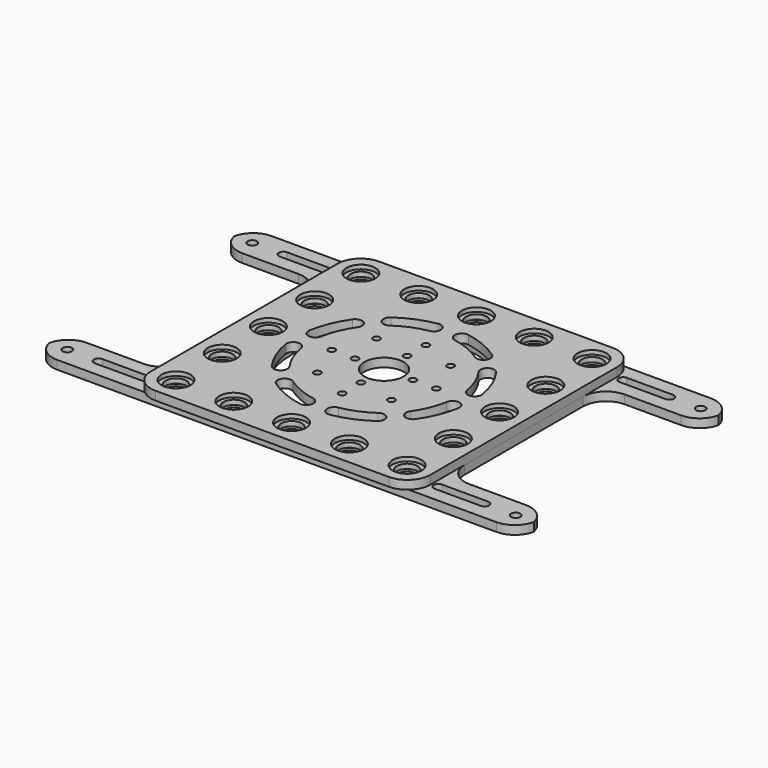
from build123d import *

# Parameters (mm, degrees)
F0_R        = 4.5
F0_W        = 24
F0_H        = 4
F0_R_2      = 2
F1_DEPTH    = 3.75
F2_T1_DEPTH = 3.75
F2_T3_DEPTH = 53.75
F3_R        = 2.5
F4_R        = 1.99999
F9_W        = 121
F9_H        = 121
F9_R        = 6.25
F9_R_2      = 1.5
F9_R_3      = 8.5
F10_DEPTH   = 3.75
F9_R_4      = 4.5
F11_DEPTH   = 2
F12_R       = 10
F6_R        = 6.25
F6_R_2      = 4.5
F13_DEPTH   = 1


# Not quite as in the source:
# - a fillet or chamfer that OpenCascade refuses, or shapes differently, is made with other operations: its cross-section is extruded or revolved along the edge and cut away or added
# - two fillets or chamfers of one size are made in one step
# - a fillet or chamfer is up to 0.001 mm smaller than in the source, because OpenCascade refuses the exact size
# - a feature names something its author has since deleted; it is built from what else it names


with BuildPart() as f1:
    # F0 (on Top) → F1 (new body)
    with BuildSketch(Plane.XY):
        with BuildLine():
            ThreePointArc((28.2842712475, 28.2842712475), (36.9551813005, 15.3073372946), (40, 0))
            ThreePointArc((40, 0), (28.2842712475, -28.2842712475), (0, -40))
            Line((0, -40), (0, -45.5))
            ThreePointArc((0, -45.5), (3.1819805153, -46.8180194847), (4.5, -50))
            ThreePointArc((4.5, -50), (3.1819805153, -53.1819805153), (0, -54.5))
            Line((0, -54.5), (0, -58))
            Line((0, -58), (105, -58))
            Line((105, -58), (105, -42))
            Line((105, -42), (60.5, -42))
            Line((60.5, -42), (60.5, 42))
            Line((60.5, 42), (105, 42))
            Line((105, 42), (105, 58))
            Line((105, 58), (0, 58))
            Line((0, 58), (0, 54.5))
            ThreePointArc((0, 54.5), (3.1819805153, 53.1819805153), (4.5, 50))
            ThreePointArc((4.5, 50), (3.1819805153, 46.8180194847), (0, 45.5))
            Line((0, 45.5), (0, 40))
            ThreePointArc((0, 40), (15.3073372946, 36.9551813005), (28.2842712475, 28.2842712475))
        make_face()
        with Locations((25, -50)):
            Circle(F0_R, mode=Mode.SUBTRACT)
        with Locations((50, -50)):
            Circle(F0_R, mode=Mode.SUBTRACT)
        Polygon((43.4109150689, -43.4109150689), (26.0242501957, -38.752172257), (38.752172257, -26.0242501957), align=None, mode=Mode.SUBTRACT)
        with Locations((73.5, -50)):
            Rectangle(F0_W, F0_H, mode=Mode.SUBTRACT)
        with Locations((97, -50)):
            Circle(F0_R_2, mode=Mode.SUBTRACT)
        with Locations((50, -25)):
            Circle(F0_R, mode=Mode.SUBTRACT)
        with Locations((50, 0)):
            Circle(F0_R, mode=Mode.SUBTRACT)
        with Locations((50, 25)):
            Circle(F0_R, mode=Mode.SUBTRACT)
        Polygon((38.752172257, 26.0242501957), (32.3882112263, 32.3882112263), (26.0242501957, 38.752172257), (43.4109150689, 43.4109150689), align=None, mode=Mode.SUBTRACT)
        with Locations((25, 50)):
            Circle(F0_R, mode=Mode.SUBTRACT)
        with Locations((50, 50)):
            Circle(F0_R, mode=Mode.SUBTRACT)
        with Locations((73.5, 50)):
            Rectangle(F0_W, F0_H, mode=Mode.SUBTRACT)
        with Locations((97, 50)):
            Circle(F0_R_2, mode=Mode.SUBTRACT)
        with BuildLine():
            Line((0, -45.5), (0, -40))
            ThreePointArc((0, -40), (-40, 0), (0, 40))
            Line((0, 40), (0, 45.5))
            ThreePointArc((0, 45.5), (-4.5, 50), (0, 54.5))
            Line((0, 54.5), (0, 58))
            Line((0, 58), (-105, 58))
            Line((-105, 58), (-105, 42))
            Line((-105, 42), (-60.5, 42))
            Line((-60.5, 42), (-60.5, -42))
            Line((-60.5, -42), (-105, -42))
            Line((-105, -42), (-105, -58))
            Line((-105, -58), (0, -58))
            Line((0, -58), (0, -54.5))
            ThreePointArc((0, -54.5), (-4.5, -50), (0, -45.5))
        make_face()
        with Locations((-97, -50)):
            Circle(F0_R_2, mode=Mode.SUBTRACT)
        with Locations((-73.5, -50)):
            Rectangle(F0_W, F0_H, mode=Mode.SUBTRACT)
        with Locations((-50, -50)):
            Circle(F0_R, mode=Mode.SUBTRACT)
        with Locations((-25, -50)):
            Circle(F0_R, mode=Mode.SUBTRACT)
        Polygon((-38.752172257, -26.0242501957), (-26.0242501957, -38.752172257), (-43.4109150689, -43.4109150689), align=None, mode=Mode.SUBTRACT)
        with Locations((-50, -25)):
            Circle(F0_R, mode=Mode.SUBTRACT)
        with Locations((-50, 0)):
            Circle(F0_R, mode=Mode.SUBTRACT)
        with Locations((-50, 25)):
            Circle(F0_R, mode=Mode.SUBTRACT)
        with Locations((-97, 50)):
            Circle(F0_R_2, mode=Mode.SUBTRACT)
        Polygon((-61.5, 52), (-61.5, 50), (-61.5, 48), (-85.5, 48), (-85.5, 50), (-85.5, 52), align=None, mode=Mode.SUBTRACT)
        Polygon((-38.752172257, 26.0242501957), (-43.4109150689, 43.4109150689), (-26.0242501957, 38.752172257), align=None, mode=Mode.SUBTRACT)
        with BuildLine():
            ThreePointArc((-54.5, 50), (-50, 54.5), (-45.5, 50))
            ThreePointArc((-45.5, 50), (-50, 45.5), (-54.5, 50))
        make_face(mode=Mode.SUBTRACT)
        with Locations((-25, 50)):
            Circle(F0_R, mode=Mode.SUBTRACT)
    extrude(amount=-F1_DEPTH)

    # F2: fillet of radius 10 on 12 edges, made by hand

    # F2_s2 → F2_t1 (join)
    with BuildSketch(Plane.XY.offset(-3.75)):
        with BuildLine():
            ThreePointArc((70.5, -42), (63.4289321881, -39.0710678119), (60.5, -32))
            Line((60.5, -32), (60.5, -42))
            Line((60.5, -42), (70.5, -42))
        make_face()
        with BuildLine():
            ThreePointArc((60.5, 32), (63.4289321881, 39.0710678119), (70.5, 42))
            Line((70.5, 42), (60.5, 42))
            Line((60.5, 42), (60.5, 32))
        make_face()
        with BuildLine():
            ThreePointArc((-70.5, 42), (-63.4289321881, 39.0710678119), (-60.5, 32))
            Line((-60.5, 32), (-60.5, 42))
            Line((-60.5, 42), (-70.5, 42))
        make_face()
        with BuildLine():
            ThreePointArc((-60.5, -32), (-63.4289321881, -39.0710678119), (-70.5, -42))
            Line((-70.5, -42), (-60.5, -42))
            Line((-60.5, -42), (-60.5, -32))
        make_face()
    extrude(amount=F2_T1_DEPTH)

    # F2_s4 → F2_t3 (cut)
    with BuildSketch(Plane.XY.offset(-28.75)):
        with BuildLine():
            ThreePointArc((-95, 58), (-102.0710678119, 55.0710678119), (-105, 48))
            Line((-105, 48), (-105, 58))
            Line((-105, 58), (-95, 58))
        make_face()
        with BuildLine():
            ThreePointArc((-105, -48), (-102.0710678119, -55.0710678119), (-95, -58))
            Line((-95, -58), (-105, -58))
            Line((-105, -58), (-105, -48))
        make_face()
        with BuildLine():
            ThreePointArc((105, 48), (102.0710678119, 55.0710678119), (95, 58))
            Line((95, 58), (105, 58))
            Line((105, 58), (105, 48))
        make_face()
        with BuildLine():
            ThreePointArc((105, -48), (102.0710678119, -55.0710678119), (95, -58))
            Line((95, -58), (105, -58))
            Line((105, -58), (105, -48))
        make_face()
        with BuildLine():
            ThreePointArc((105, -52), (102.0710678119, -44.9289321881), (95, -42))
            Line((95, -42), (105, -42))
            Line((105, -42), (105, -52))
        make_face()
        with BuildLine():
            ThreePointArc((95, 42), (102.0710678119, 44.9289321881), (105, 52))
            Line((105, 52), (105, 42))
            Line((105, 42), (95, 42))
        make_face()
        with BuildLine():
            ThreePointArc((-105, 52), (-102.0710678119, 44.9289321881), (-95, 42))
            Line((-95, 42), (-105, 42))
            Line((-105, 42), (-105, 52))
        make_face()
        with BuildLine():
            ThreePointArc((-95, -42), (-102.0710678119, -44.9289321881), (-105, -52))
            Line((-105, -52), (-105, -42))
            Line((-105, -42), (-95, -42))
        make_face()
    extrude(amount=F2_T3_DEPTH, mode=Mode.SUBTRACT)

    # F3
    f3_edges = [f1.edges().sort_by_distance(p)[0] for p in [
        (-38.752172, 26.02425, -1.875),
        (-43.410915, 43.410915, -1.875),
        (-26.02425, 38.752172, -1.875),
        (-38.752172, -26.02425, -1.875),
        (38.752172, -26.02425, -1.875),
        (43.410915, 43.410915, -1.875),
        (38.752172, 26.02425, -1.875),
        (43.410915, -43.410915, -1.875),
        (-43.410915, -43.410915, -1.875),
        (26.02425, 38.752172, -1.875),
        (26.02425, -38.752172, -1.875),
        (-26.02425, -38.752172, -1.875),
    ]]
    fillet(f3_edges, radius=F3_R)

    # F4 (radius 2 in the source; OpenCascade refuses exactly that, so slightly less here)
    f4_edges = [f1.edges().sort_by_distance(p)[0] for p in [
        (-85.5, 52, -1.875),
        (-61.5, 52, -1.875),
        (-61.5, 48, -1.875),
        (-85.5, 48, -1.875),
        (-85.5, -48, -1.875),
        (61.5, 52, -1.875),
        (61.5, -48, -1.875),
        (85.5, -48, -1.875),
        (-61.5, -48, -1.875),
        (85.5, 52, -1.875),
        (-85.5, -52, -1.875),
        (61.5, 48, -1.875),
        (61.5, -52, -1.875),
        (-61.5, -52, -1.875),
        (85.5, -52, -1.875),
        (85.5, 48, -1.875),
    ]]
    fillet(f4_edges, radius=F4_R)

    # F6 (on Top) → F13 (cut)
    with BuildSketch(Plane.XY):
        with Locations((50, 50)):
            Circle(F6_R)
        with Locations((50, 50)):
            Circle(F6_R_2, mode=Mode.SUBTRACT)
        with Locations((50, 25)):
            Circle(F6_R)
        with Locations((50, 25)):
            Circle(F6_R_2, mode=Mode.SUBTRACT)
        with Locations((50, 0)):
            Circle(F6_R)
        with Locations((50, 0)):
            Circle(F6_R_2, mode=Mode.SUBTRACT)
        with Locations((50, -25)):
            Circle(F6_R)
        with Locations((50, -25)):
            Circle(F6_R_2, mode=Mode.SUBTRACT)
        with Locations((50, -50)):
            Circle(F6_R)
        with Locations((50, -50)):
            Circle(F6_R_2, mode=Mode.SUBTRACT)
        with Locations((25, -50)):
            Circle(F6_R)
        with Locations((25, -50)):
            Circle(F6_R_2, mode=Mode.SUBTRACT)
        with Locations((0, -50)):
            Circle(F6_R)
        with Locations((0, -50)):
            Circle(F6_R_2, mode=Mode.SUBTRACT)
        with Locations((-25, -50)):
            Circle(F6_R)
        with Locations((-25, -50)):
            Circle(F6_R_2, mode=Mode.SUBTRACT)
        with Locations((-50, -50)):
            Circle(F6_R)
        with Locations((-50, -50)):
            Circle(F6_R_2, mode=Mode.SUBTRACT)
        with Locations((-50, -25)):
            Circle(F6_R)
        with Locations((-50, -25)):
            Circle(F6_R_2, mode=Mode.SUBTRACT)
        with Locations((-50, 0)):
            Circle(F6_R)
        with Locations((-50, 0)):
            Circle(F6_R_2, mode=Mode.SUBTRACT)
        with Locations((-50, 25)):
            Circle(F6_R)
        with Locations((-50, 25)):
            Circle(F6_R_2, mode=Mode.SUBTRACT)
        with Locations((-50, 50)):
            Circle(F6_R)
        with Locations((-50, 50)):
            Circle(F6_R_2, mode=Mode.SUBTRACT)
        with Locations((-25, 50)):
            Circle(F6_R)
        with Locations((-25, 50)):
            Circle(F6_R_2, mode=Mode.SUBTRACT)
        with Locations((0, 50)):
            Circle(F6_R)
        with Locations((0, 50)):
            Circle(F6_R_2, mode=Mode.SUBTRACT)
        with Locations((25, 50)):
            Circle(F6_R)
        with Locations((25, 50)):
            Circle(F6_R_2, mode=Mode.SUBTRACT)
    extrude(amount=-F13_DEPTH, mode=Mode.SUBTRACT)


with BuildPart() as f10:
    # F9 (on Top) → F10 (new body)
    with BuildSketch(Plane.XY):
        Rectangle(F9_W, F9_H)
        with Locations((-50, -50)):
            Circle(F9_R, mode=Mode.SUBTRACT)
        with Locations((-25, -50)):
            Circle(F9_R, mode=Mode.SUBTRACT)
        with BuildLine():
            ThreePointArc((-21.8659925642, -31.0785837705), (-22.5933023963, -26.8987487967), (-18.4134674225, -26.1714389647))
            ThreePointArc((-18.4134674225, -26.1714389647), (-12.2458698357, -29.5641450404), (-5.4857142857, -31.5262896449))
            ThreePointArc((-5.4857142857, -31.5262896449), (-3.0444103458, -34.9961650134), (-6.5142857143, -37.4374689533))
            ThreePointArc((-6.5142857143, -37.4374689533), (-14.5419704299, -35.1074222354), (-21.8659925642, -31.0785837705))
        make_face(mode=Mode.SUBTRACT)
        with Locations((-50, -25)):
            Circle(F9_R, mode=Mode.SUBTRACT)
        with BuildLine():
            ThreePointArc((-31.0785837705, -21.8659925642), (-35.1074222354, -14.5419704299), (-37.4374689533, -6.5142857143))
            ThreePointArc((-37.4374689533, -6.5142857143), (-34.9961650134, -3.0444103458), (-31.5262896449, -5.4857142857))
            ThreePointArc((-31.5262896449, -5.4857142857), (-29.5641450404, -12.2458698357), (-26.1714389647, -18.4134674225))
            ThreePointArc((-26.1714389647, -18.4134674225), (-26.8987487967, -22.5933023963), (-31.0785837705, -21.8659925642))
        make_face(mode=Mode.SUBTRACT)
        with Locations((-16, -16)):
            Circle(F9_R_2, mode=Mode.SUBTRACT)
        with Locations((0, -50)):
            Circle(F9_R, mode=Mode.SUBTRACT)
        with Locations((25, -50)):
            Circle(F9_R, mode=Mode.SUBTRACT)
        with BuildLine():
            ThreePointArc((21.8659925642, -31.0785837705), (14.5419704299, -35.1074222354), (6.5142857143, -37.4374689533))
            ThreePointArc((6.5142857143, -37.4374689533), (3.0444103458, -34.9961650134), (5.4857142857, -31.5262896449))
            ThreePointArc((5.4857142857, -31.5262896449), (12.2458698357, -29.5641450404), (18.4134674225, -26.1714389647))
            ThreePointArc((18.4134674225, -26.1714389647), (22.5933023963, -26.8987487967), (21.8659925642, -31.0785837705))
        make_face(mode=Mode.SUBTRACT)
        with Locations((50, -50)):
            Circle(F9_R, mode=Mode.SUBTRACT)
        with Locations((0, -22.627416998)):
            Circle(F9_R_2, mode=Mode.SUBTRACT)
        with Locations((16, -16)):
            Circle(F9_R_2, mode=Mode.SUBTRACT)
        with Locations((0, -12.5)):
            Circle(F9_R_2, mode=Mode.SUBTRACT)
        with Locations((50, -25)):
            Circle(F9_R, mode=Mode.SUBTRACT)
        with BuildLine():
            ThreePointArc((37.4374689533, -6.5142857143), (35.1074222354, -14.5419704299), (31.0785837705, -21.8659925642))
            ThreePointArc((31.0785837705, -21.8659925642), (26.8987487967, -22.5933023963), (26.1714389647, -18.4134674225))
            ThreePointArc((26.1714389647, -18.4134674225), (29.5641450404, -12.2458698357), (31.5262896449, -5.4857142857))
            ThreePointArc((31.5262896449, -5.4857142857), (34.9961650134, -3.0444103458), (37.4374689533, -6.5142857143))
        make_face(mode=Mode.SUBTRACT)
        with Locations((-50, 0)):
            Circle(F9_R, mode=Mode.SUBTRACT)
        with BuildLine():
            ThreePointArc((-37.4374689533, 6.5142857143), (-35.1074222354, 14.5419704299), (-31.0785837705, 21.8659925642))
            ThreePointArc((-31.0785837705, 21.8659925642), (-26.8987487967, 22.5933023963), (-26.1714389647, 18.4134674225))
            ThreePointArc((-26.1714389647, 18.4134674225), (-29.5641450404, 12.2458698357), (-31.5262896449, 5.4857142857))
            ThreePointArc((-31.5262896449, 5.4857142857), (-34.9961650134, 3.0444103458), (-37.4374689533, 6.5142857143))
        make_face(mode=Mode.SUBTRACT)
        with Locations((-50, 25)):
            Circle(F9_R, mode=Mode.SUBTRACT)
        with Locations((-22.627416998, 0)):
            Circle(F9_R_2, mode=Mode.SUBTRACT)
        with Locations((-12.5, 0)):
            Circle(F9_R_2, mode=Mode.SUBTRACT)
        with Locations((-16, 16)):
            Circle(F9_R_2, mode=Mode.SUBTRACT)
        with Locations((-50, 50)):
            Circle(F9_R, mode=Mode.SUBTRACT)
        with BuildLine():
            ThreePointArc((-6.5142857143, 37.4374689533), (-3.0444103458, 34.9961650134), (-5.4857142857, 31.5262896449))
            ThreePointArc((-5.4857142857, 31.5262896449), (-12.2458698357, 29.5641450404), (-18.4134674225, 26.1714389647))
            ThreePointArc((-18.4134674225, 26.1714389647), (-22.5933023963, 26.8987487967), (-21.8659925642, 31.0785837705))
            ThreePointArc((-21.8659925642, 31.0785837705), (-14.5419704299, 35.1074222354), (-6.5142857143, 37.4374689533))
        make_face(mode=Mode.SUBTRACT)
        with Locations((-25, 50)):
            Circle(F9_R, mode=Mode.SUBTRACT)
        Circle(F9_R_3, mode=Mode.SUBTRACT)
        with Locations((12.5, 0)):
            Circle(F9_R_2, mode=Mode.SUBTRACT)
        with Locations((0, 12.5)):
            Circle(F9_R_2, mode=Mode.SUBTRACT)
        with Locations((22.627416998, 0)):
            Circle(F9_R_2, mode=Mode.SUBTRACT)
        with Locations((0, 22.627416998)):
            Circle(F9_R_2, mode=Mode.SUBTRACT)
        with Locations((16, 16)):
            Circle(F9_R_2, mode=Mode.SUBTRACT)
        with BuildLine():
            ThreePointArc((31.5262896449, 5.4857142857), (29.5641450404, 12.2458698357), (26.1714389647, 18.4134674225))
            ThreePointArc((26.1714389647, 18.4134674225), (26.8987487967, 22.5933023963), (31.0785837705, 21.8659925642))
            ThreePointArc((31.0785837705, 21.8659925642), (35.1074222354, 14.5419704299), (37.4374689533, 6.5142857143))
            ThreePointArc((37.4374689533, 6.5142857143), (34.9961650134, 3.0444103458), (31.5262896449, 5.4857142857))
        make_face(mode=Mode.SUBTRACT)
        with Locations((50, 0)):
            Circle(F9_R, mode=Mode.SUBTRACT)
        with Locations((50, 25)):
            Circle(F9_R, mode=Mode.SUBTRACT)
        with BuildLine():
            ThreePointArc((18.4134674225, 26.1714389647), (12.2458698357, 29.5641450404), (5.4857142857, 31.5262896449))
            ThreePointArc((5.4857142857, 31.5262896449), (3.0444103458, 34.9961650134), (6.5142857143, 37.4374689533))
            ThreePointArc((6.5142857143, 37.4374689533), (14.5419704299, 35.1074222354), (21.8659925642, 31.0785837705))
            ThreePointArc((21.8659925642, 31.0785837705), (22.5933023963, 26.8987487967), (18.4134674225, 26.1714389647))
        make_face(mode=Mode.SUBTRACT)
        with Locations((0, 50)):
            Circle(F9_R, mode=Mode.SUBTRACT)
        with Locations((25, 50)):
            Circle(F9_R, mode=Mode.SUBTRACT)
        with Locations((50, 50)):
            Circle(F9_R, mode=Mode.SUBTRACT)
    extrude(amount=F10_DEPTH)

    # F9 (on Top) → F11 (join)
    with BuildSketch(Plane.XY):
        with Locations((-50, 50)):
            Circle(F9_R)
        with Locations((-50, 50)):
            Circle(F9_R_4, mode=Mode.SUBTRACT)
        with Locations((-25, 50)):
            Circle(F9_R)
        with Locations((-25, 50)):
            Circle(F9_R_4, mode=Mode.SUBTRACT)
        with Locations((0, 50)):
            Circle(F9_R)
        with Locations((0, 50)):
            Circle(F9_R_4, mode=Mode.SUBTRACT)
        with Locations((25, 50)):
            Circle(F9_R)
        with Locations((25, 50)):
            Circle(F9_R_4, mode=Mode.SUBTRACT)
        with Locations((50, 50)):
            Circle(F9_R)
        with Locations((50, 50)):
            Circle(F9_R_4, mode=Mode.SUBTRACT)
        with Locations((-50, 25)):
            Circle(F9_R)
        with Locations((-50, 25)):
            Circle(F9_R_4, mode=Mode.SUBTRACT)
        with Locations((50, 25)):
            Circle(F9_R)
        with Locations((50, 25)):
            Circle(F9_R_4, mode=Mode.SUBTRACT)
        with Locations((50, 0)):
            Circle(F9_R)
        with Locations((50, 0)):
            Circle(F9_R_4, mode=Mode.SUBTRACT)
        with Locations((50, -25)):
            Circle(F9_R)
        with Locations((50, -25)):
            Circle(F9_R_4, mode=Mode.SUBTRACT)
        with Locations((50, -50)):
            Circle(F9_R)
        with Locations((50, -50)):
            Circle(F9_R_4, mode=Mode.SUBTRACT)
        with Locations((25, -50)):
            Circle(F9_R)
        with Locations((25, -50)):
            Circle(F9_R_4, mode=Mode.SUBTRACT)
        with Locations((0, -50)):
            Circle(F9_R)
        with Locations((0, -50)):
            Circle(F9_R_4, mode=Mode.SUBTRACT)
        with Locations((-25, -50)):
            Circle(F9_R)
        with Locations((-25, -50)):
            Circle(F9_R_4, mode=Mode.SUBTRACT)
        with Locations((-50, -50)):
            Circle(F9_R)
        with Locations((-50, -50)):
            Circle(F9_R_4, mode=Mode.SUBTRACT)
        with Locations((-50, -25)):
            Circle(F9_R)
        with Locations((-50, -25)):
            Circle(F9_R_4, mode=Mode.SUBTRACT)
        with Locations((-50, 0)):
            Circle(F9_R)
        with Locations((-50, 0)):
            Circle(F9_R_4, mode=Mode.SUBTRACT)
    extrude(amount=F11_DEPTH)

    # F12
    f12_edges = [f10.edges().sort_by_distance(p)[0] for p in [
        (60.5, 60.5, 1.875),
        (-60.5, 60.5, 1.875),
        (60.5, -60.5, 1.875),
        (-60.5, -60.5, 1.875),
    ]]
    fillet(f12_edges, radius=F12_R)


solid = Compound([f1.part, f10.part])
